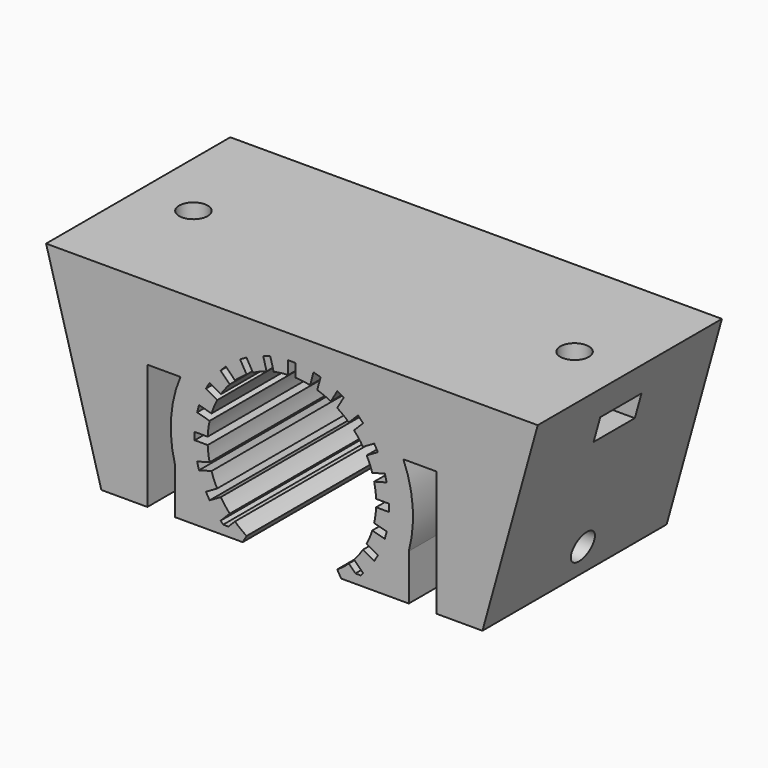
from build123d import *

# Parameters (mm, degrees)
F1_DEPTH  = 25
F2_W      = 3.2
F2_H      = 0.8
F2_W_2    = 0.8
F2_H_2    = 3.2
F3_DEPTH  = 25.001
F4_SIZE   = 0.4
F5_R      = 1.55
F6_DEPTH  = 11.001
F7_DEPTH  = 2.6
F8_R      = 1.6
F9_DEPTH  = 0.3
F10_SIZE  = 0.1
F11_R     = 1.55
F12_DEPTH = 7
F15_W     = 5.6
F15_H     = 2.6
F16_DEPTH = 10


# Not quite as in the source:
# - a pattern or mirror of a feature is missing from the dataset's text; its kind, count and spacing are read off the source's solid


with BuildPart() as f1:
    # F0 (on Front) → F1 (new body)
    with BuildSketch(Plane.XZ):
        with BuildLine():
            Line((26.6893656264, 13.15), (0, 13.15))
            Line((0, 13.15), (-26.6893656264, 13.15))
            Line((-26.6893656264, 13.15), (-20.6893656264, -8.45))
            Line((-20.6893656264, -8.45), (-15.6893656264, -8.45))
            Line((-15.6893656264, -8.45), (-15.6893656264, 5.15))
            Line((-15.6893656264, 5.15), (-12.0995867698, 5.15))
            ThreePointArc((-12.0995867698, 5.15), (-13.1191859589, 0.8996998249), (-12.6893656264, -3.45))
            Line((-12.6893656264, -3.45), (-12.6893656264, -8.45))
            Line((-12.6893656264, -8.45), (-3.509985755, -8.45))
            ThreePointArc((-3.509985755, -8.45), (-8.9732937097, 1.7895530168), (0, 9.15))
            ThreePointArc((0, 9.15), (8.9732937097, 1.7895530168), (3.509985755, -8.45))
            Line((3.509985755, -8.45), (12.6893656264, -8.45))
            Line((12.6893656264, -8.45), (12.6893656264, -3.45))
            ThreePointArc((12.6893656264, -3.45), (13.1191859589, 0.8996998249), (12.0995867698, 5.15))
            Line((12.0995867698, 5.15), (15.6893656264, 5.15))
            Line((15.6893656264, 5.15), (15.6893656264, -8.45))
            Line((15.6893656264, -8.45), (20.6893656264, -8.45))
            Line((20.6893656264, -8.45), (26.6893656264, 13.15))
        make_face()
    extrude(amount=F1_DEPTH)

    # F2 (on face) → F3 (cut, through all)
    with BuildSketch(Plane(origin=(0, 0, 0), x_dir=(-1, 0, 0), z_dir=(0, 1, 0))):
        with Locations((-8.95, 0)):
            Rectangle(F2_W, F2_H)
        Polygon((-7.2030824413, -1.515949651), (-10.2940450854, -2.3441705953), (-10.0869898493, -3.1169112563), (-6.9960272052, -2.288690312), align=None)
        Polygon((-6.5652867178, -3.3285898385), (-9.3365680099, -4.9285898385), (-8.9365680099, -5.6214101615), (-6.1652867178, -4.0214101615), align=None)
        Polygon((-5.4800775542, -4.9143921292), (-7.742819254, -7.177133829), (-7.177133829, -7.742819254), (-4.9143921292, -5.4800775542), align=None)
        Polygon((-4.0214101615, -6.1652867178), (-5.6214101615, -8.9365680099), (-4.9285898385, -9.3365680099), (-3.3285898385, -6.5652867178), align=None)
        Polygon((-3.3285898385, -6.5652867178), (-4.9285898385, -9.3365680099), (-3.1169112563, -10.0869898493), (-2.288690312, -6.9960272052), align=None)
        Polygon((-2.288690312, -6.9960272052), (-3.1169112563, -10.0869898493), (-2.3441705953, -10.2940450854), (-1.515949651, -7.2030824413), align=None)
        with Locations((0, -8.95)):
            Rectangle(F2_W_2, F2_H_2)
        Polygon((1.515949651, -7.2030824413), (2.3441705953, -10.2940450854), (3.1169112563, -10.0869898493), (2.288690312, -6.9960272052), align=None)
        Polygon((2.288690312, -6.9960272052), (3.1169112563, -10.0869898493), (4.9285898385, -9.3365680099), (3.3285898385, -6.5652867178), align=None)
        Polygon((3.3285898385, -6.5652867178), (4.9285898385, -9.3365680099), (5.6214101615, -8.9365680099), (4.0214101615, -6.1652867178), align=None)
        Polygon((4.9143921292, -5.4800775542), (7.177133829, -7.742819254), (7.742819254, -7.177133829), (5.4800775542, -4.9143921292), align=None)
        Polygon((6.1652867178, -4.0214101615), (8.9365680099, -5.6214101615), (9.3365680099, -4.9285898385), (6.5652867178, -3.3285898385), align=None)
        Polygon((6.9960272052, -2.288690312), (10.0869898493, -3.1169112563), (10.2940450854, -2.3441705953), (7.2030824413, -1.515949651), align=None)
        with Locations((8.95, 0)):
            Rectangle(F2_W, F2_H)
        Polygon((7.2030824413, 1.515949651), (10.2940450854, 2.3441705953), (10.0869898493, 3.1169112563), (6.9960272052, 2.288690312), align=None)
        Polygon((6.5652867178, 3.3285898385), (9.3365680099, 4.9285898385), (8.9365680099, 5.6214101615), (6.1652867178, 4.0214101615), align=None)
        Polygon((5.4800775542, 4.9143921292), (7.742819254, 7.177133829), (7.177133829, 7.742819254), (4.9143921292, 5.4800775542), align=None)
        Polygon((4.0214101615, 6.1652867178), (5.6214101615, 8.9365680099), (4.9285898385, 9.3365680099), (3.3285898385, 6.5652867178), align=None)
        Polygon((2.288690312, 6.9960272052), (3.1169112563, 10.0869898493), (2.3441705953, 10.2940450854), (1.515949651, 7.2030824413), align=None)
        with Locations((0, 8.95)):
            Rectangle(F2_W_2, F2_H_2)
        Polygon((-1.515949651, 7.2030824413), (-2.3441705953, 10.2940450854), (-3.1169112563, 10.0869898493), (-2.288690312, 6.9960272052), align=None)
        Polygon((-3.3285898385, 6.5652867178), (-4.9285898385, 9.3365680099), (-5.6214101615, 8.9365680099), (-4.0214101615, 6.1652867178), align=None)
        Polygon((-4.9143921292, 5.4800775542), (-7.177133829, 7.742819254), (-7.742819254, 7.177133829), (-5.4800775542, 4.9143921292), align=None)
        Polygon((-6.1652867178, 4.0214101615), (-8.9365680099, 5.6214101615), (-9.3365680099, 4.9285898385), (-6.5652867178, 3.3285898385), align=None)
        Polygon((-6.9960272052, 2.288690312), (-10.0869898493, 3.1169112563), (-10.2940450854, 2.3441705953), (-7.2030824413, 1.515949651), align=None)
    extrude(amount=-F3_DEPTH, mode=Mode.SUBTRACT)

    # F4
    f4_edges = [f1.edges().sort_by_distance(p)[0] for p in [
        (7.177134, -12.5, -7.742819),
        (-7.177134, -12.5, -7.742819),
    ]]
    chamfer(f4_edges, length=F4_SIZE)

    # F5 (on face) → F6 (cut, through all)
    with BuildSketch(Plane.YZ.offset(-15.6893656264)):
        with Locations((-12.5, -5.2)):
            Circle(F5_R)
    f6 = extrude(amount=-F6_DEPTH, mode=Mode.SUBTRACT)

    # F6_copies: F6 across plane
    add(f6.mirror(Plane(origin=(-1e-06, 0, 0), x_dir=(0, 0, 1), z_dir=(1, 0, 0))), mode=Mode.SUBTRACT)

    # F5 (on face) → F7 (cut)
    with BuildSketch(Plane.YZ.offset(-15.6893656264)):
        Polygon((-14.0877132403, -7.95), (-10.9122867597, -7.95), (-9.3245735195, -5.2), (-10.9122867597, -2.45), (-14.0877132403, -2.45), (-15.6754264805, -5.2), align=None)
        with Locations((-12.5, -5.2)):
            Circle(F5_R, mode=Mode.SUBTRACT)
    f7 = extrude(amount=-F7_DEPTH, mode=Mode.SUBTRACT)

    # F7_copies: F7 across plane
    add(f7.mirror(Plane(origin=(0, 0, 0), x_dir=(0, 0, 1), z_dir=(1, 0, 0))), mode=Mode.SUBTRACT)

    # F8 (on face) → F9 (cut)
    with BuildSketch(Plane(origin=(-12.6893656264, 0, 0), x_dir=(0, -1, 0), z_dir=(-1, 0, 0))):
        with Locations((12.5, -5.2)):
            Circle(F8_R)
    f9 = extrude(amount=-F9_DEPTH, mode=Mode.SUBTRACT)

    # F9_copies: F9 across plane
    add(f9.mirror(Plane(origin=(0, 0, 0), x_dir=(0, 0, 1), z_dir=(1, 0, 0))), mode=Mode.SUBTRACT)

    # F10
    f10_edges = [f1.edges().sort_by_distance(p)[0] for p in [
        (-12.689366, -10.9, -5.2),
        (-12.389366, -10.9, -5.2),
        (12.689366, -10.9, -5.2),
        (12.389366, -10.9, -5.2),
    ]]
    chamfer(f10_edges, length=F10_SIZE)

    # F11 (on face) → F12 (cut)
    with BuildSketch(Plane.XY.offset(13.15)):
        with Locations((-20.6893656264, -12.5)):
            Circle(F11_R)
    f12 = extrude(amount=-F12_DEPTH, mode=Mode.SUBTRACT)

    # F12_copies: F12 across plane
    add(f12.mirror(Plane(origin=(0, 0, 0), x_dir=(0, 0, 1), z_dir=(1, 0, 0))), mode=Mode.SUBTRACT)

    # F15 (on plane+point) → F16 (cut)
    with BuildSketch(Plane.YZ.offset(-26.6893656264)):
        with Locations((-12.5, 8.35)):
            Rectangle(F15_W, F15_H)
    f16 = extrude(amount=F16_DEPTH, mode=Mode.SUBTRACT)

    # F16_copies: F16 across plane
    add(f16.mirror(Plane(origin=(0, 0, 0), x_dir=(0, 0, 1), z_dir=(1, 0, 0))), mode=Mode.SUBTRACT)


solid = f1.part
